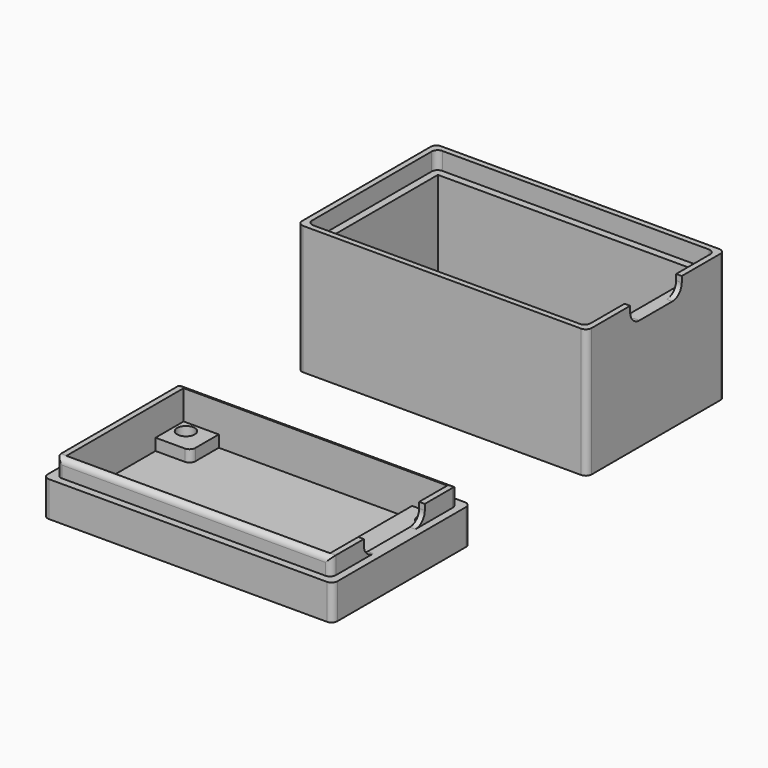
from build123d import *

# Parameters (mm, degrees)
F1_DEPTH     = 2
F0_W         = 6
F0_H         = 6
F0_H_2       = 25
F2_DEPTH     = 4
F0_W_2       = 49.44
F0_H_3       = 29.44
F3_DEPTH     = 6
F4_D         = 3
F5_W         = 46.92
F5_H         = 26.92
F5_W_2       = 45
F5_H_2       = 25
F6_DEPTH     = 3
F7_W         = 0.96
F7_H         = 13
F8_DEPTH     = 3
F0_W_3       = 45
F9_DEPTH     = 2
F10_DEPTH    = 19
F11_W        = 49.44
F11_H        = 29.44
F11_W_2      = 47.52
F11_H_2      = 27.52
F12_DEPTH    = 3
F13_T1_DEPTH = 4.5
F13_T3_DEPTH = 5.5
F13_T5_DEPTH = 51.92
F13_T7_DEPTH = 11
F13_2_F1_R   = 1
F13_2_F2_R   = 1
F14_W        = 0.96
F14_H        = 11
F15_DEPTH    = 3
F16_R        = 2
F16_2_R      = 2


# Not quite as in the source:
# - a fillet or chamfer that OpenCascade refuses, or shapes differently, is made with other operations: its cross-section is extruded or revolved along the edge and cut away or added


with BuildPart() as f1:
    # F0 (on Top) → F1 (new body)
    with BuildSketch(Plane.XY):
        Polygon((-16.5, -12.5), (16.5, -12.5), (16.5, 12.5), (-16.5, 12.5), (-16.5, 6.5), (-22.5, 6.5), (-22.5, -6.5), (-16.5, -6.5), align=None)
    extrude(amount=F1_DEPTH)

    # F0 (on Top) → F2 (join)
    with BuildSketch(Plane.XY):
        with Locations((-19.5, 9.5)):
            Rectangle(F0_W, F0_H)
        with Locations((-19.5, -9.5)):
            Rectangle(F0_W, F0_H)
        with Locations((19.5, 0)):
            Rectangle(F0_W, F0_H_2)
    extrude(amount=F2_DEPTH)

    # F0 (on Top) → F3 (join)
    with BuildSketch(Plane.XY):
        Rectangle(F0_W_2, F0_H_3)
        Polygon((22.5, 12.5), (22.5, -12.5), (16.5, -12.5), (-16.5, -12.5), (-22.5, -12.5), (-22.5, -6.5), (-22.5, 6.5), (-22.5, 12.5), (-16.5, 12.5), (16.5, 12.5), align=None, mode=Mode.SUBTRACT)
    extrude(amount=F3_DEPTH)

    # F4 (through all)
    with Locations(Plane(origin=(0, 0, 0), x_dir=(1, 0, 0), z_dir=(0, 0, -1))):
        with Locations((-20.5, 10.5), (20.5, -10.5), (20.5, 10.5), (-20.5, -10.5)):
            Hole(F4_D / 2)

    # F5 (on face) → F6 (join)
    with BuildSketch(Plane.XY.offset(6)):
        Rectangle(F5_W, F5_H)
        Rectangle(F5_W_2, F5_H_2, mode=Mode.SUBTRACT)
    extrude(amount=F6_DEPTH)

    # F7 (on face) → F8 (cut)
    with BuildSketch(Plane.XY.offset(9)):
        with Locations((22.98, 0)):
            Rectangle(F7_W, F7_H)
    extrude(amount=-F8_DEPTH, mode=Mode.SUBTRACT)

    # F13: fillet of radius 1 on 12 edges, made by hand

    # F13_s2 → F13_t1 (cut)
    with BuildSketch(Plane.XY.offset(2)):
        with BuildLine():
            ThreePointArc((-16.5, 7.5), (-16.7928932188, 6.7928932188), (-17.5, 6.5))
            Line((-17.5, 6.5), (-16.5, 6.5))
            Line((-16.5, 6.5), (-16.5, 7.5))
        make_face()
        with BuildLine():
            ThreePointArc((-17.5, -6.5), (-16.7928932188, -6.7928932188), (-16.5, -7.5))
            Line((-16.5, -7.5), (-16.5, -6.5))
            Line((-16.5, -6.5), (-17.5, -6.5))
        make_face()
    extrude(amount=F13_T1_DEPTH, mode=Mode.SUBTRACT)

    # F13_s4 → F13_t3 (cut)
    with BuildSketch(Plane.XY.offset(6)):
        with BuildLine():
            ThreePointArc((-23.46, 12.46), (-23.1671067812, 13.1671067812), (-22.46, 13.46))
            Line((-22.46, 13.46), (-23.46, 13.46))
            Line((-23.46, 13.46), (-23.46, 12.46))
        make_face()
        with BuildLine():
            ThreePointArc((22.46, 13.46), (23.1671067812, 13.1671067812), (23.46, 12.46))
            Line((23.46, 12.46), (23.46, 13.46))
            Line((23.46, 13.46), (22.46, 13.46))
        make_face()
        with BuildLine():
            ThreePointArc((-22.46, -13.46), (-23.1671067812, -13.1671067812), (-23.46, -12.46))
            Line((-23.46, -12.46), (-23.46, -13.46))
            Line((-23.46, -13.46), (-22.46, -13.46))
        make_face()
        with BuildLine():
            ThreePointArc((22.46, -13.46), (23.1671067812, -13.1671067812), (23.46, -12.46))
            Line((23.46, -12.46), (23.46, -13.46))
            Line((23.46, -13.46), (22.46, -13.46))
        make_face()
    extrude(amount=F13_T3_DEPTH, mode=Mode.SUBTRACT)

    # F13_s6 → F13_t5 (cut)
    with BuildSketch(Plane.YZ.offset(-25.96)):
        with BuildLine():
            ThreePointArc((-12.46, 9), (-13.1671067812, 8.7071067812), (-13.46, 8))
            Line((-13.46, 8), (-13.46, 9))
            Line((-13.46, 9), (-12.46, 9))
        make_face()
        with BuildLine():
            ThreePointArc((12.46, 9), (13.1671067812, 8.7071067812), (13.46, 8))
            Line((13.46, 8), (13.46, 9))
            Line((13.46, 9), (12.46, 9))
        make_face()
    extrude(amount=F13_T5_DEPTH, mode=Mode.SUBTRACT)

    # F13_s8 → F13_t7 (cut)
    with BuildSketch(Plane.XY.offset(-2.5)):
        with BuildLine():
            ThreePointArc((-23.72, -14.72), (-24.4271067812, -14.4271067812), (-24.72, -13.72))
            Line((-24.72, -13.72), (-24.72, -14.72))
            Line((-24.72, -14.72), (-23.72, -14.72))
        make_face()
        with BuildLine():
            ThreePointArc((-23.72, 14.72), (-24.4271067812, 14.4271067812), (-24.72, 13.72))
            Line((-24.72, 13.72), (-24.72, 14.72))
            Line((-24.72, 14.72), (-23.72, 14.72))
        make_face()
        with BuildLine():
            ThreePointArc((24.72, -13.72), (24.4271067812, -14.4271067812), (23.72, -14.72))
            Line((23.72, -14.72), (24.72, -14.72))
            Line((24.72, -14.72), (24.72, -13.72))
        make_face()
        with BuildLine():
            ThreePointArc((24.72, 13.72), (24.4271067812, 14.4271067812), (23.72, 14.72))
            Line((23.72, 14.72), (24.72, 14.72))
            Line((24.72, 14.72), (24.72, 13.72))
        make_face()
    extrude(amount=F13_T7_DEPTH, mode=Mode.SUBTRACT)

    # F16
    f16_edges = [f1.edges().sort_by_distance(p)[0] for p in [
        (22.98, 6.5, 6),
        (22.98, -6.5, 6),
    ]]
    fillet(f16_edges, radius=F16_R)


with BuildPart() as f9:
    # F0 (on Top) → F9 (new body)
    with BuildSketch(Plane.XY):
        with Locations((0, 54.2441010475)):
            Rectangle(F0_W_3, F0_H_2)
    extrude(amount=F9_DEPTH)

    # F0 (on Top) → F10 (join)
    with BuildSketch(Plane.XY):
        with Locations((0, 54.2441010475)):
            Rectangle(F0_W_2, F0_H_3)
        with Locations((0, 54.2441010475)):
            Rectangle(F0_W_3, F0_H_2, mode=Mode.SUBTRACT)
    extrude(amount=F10_DEPTH)

    # F11 (on face) → F12 (join)
    with BuildSketch(Plane.XY.offset(19)):
        with Locations((0, 54.2441010475)):
            Rectangle(F11_W, F11_H)
        with Locations((0, 54.2441010475)):
            Rectangle(F11_W_2, F11_H_2, mode=Mode.SUBTRACT)
    extrude(amount=F12_DEPTH)

    # F13#2: fillet of radius 1 on 8 edges, made by hand

    # F13_2_f1
    f13_2_f1_edges = [f9.edges().sort_by_distance(p)[0] for p in [
        (-23.76, 68.0041010475, 20.5),
        (23.76, 68.0041010475, 20.5),
        (23.76, 40.4841010475, 20.5),
        (-23.76, 40.4841010475, 20.5),
    ]]
    fillet(f13_2_f1_edges, radius=F13_2_F1_R)

    # F13_2_f2
    f13_2_f2_edges = [f9.edges().sort_by_distance(p)[0] for p in [
        (-24.72, 39.5241010475, 11),
        (-24.72, 68.9641010475, 11),
        (24.72, 68.9641010475, 11),
        (24.72, 39.5241010475, 11),
    ]]
    fillet(f13_2_f2_edges, radius=F13_2_F2_R)

    # F14 (on face) → F15 (cut)
    with BuildSketch(Plane.XY.offset(22)):
        with Locations((24.24, 54.2441010475)):
            Rectangle(F14_W, F14_H)
    extrude(amount=-F15_DEPTH, mode=Mode.SUBTRACT)

    # F16#2
    f16_2_edges = [f9.edges().sort_by_distance(p)[0] for p in [
        (24.24, 59.744101, 19),
        (24.24, 48.744101, 19),
    ]]
    fillet(f16_2_edges, radius=F16_2_R)


solid = Compound([f1.part, f9.part])
